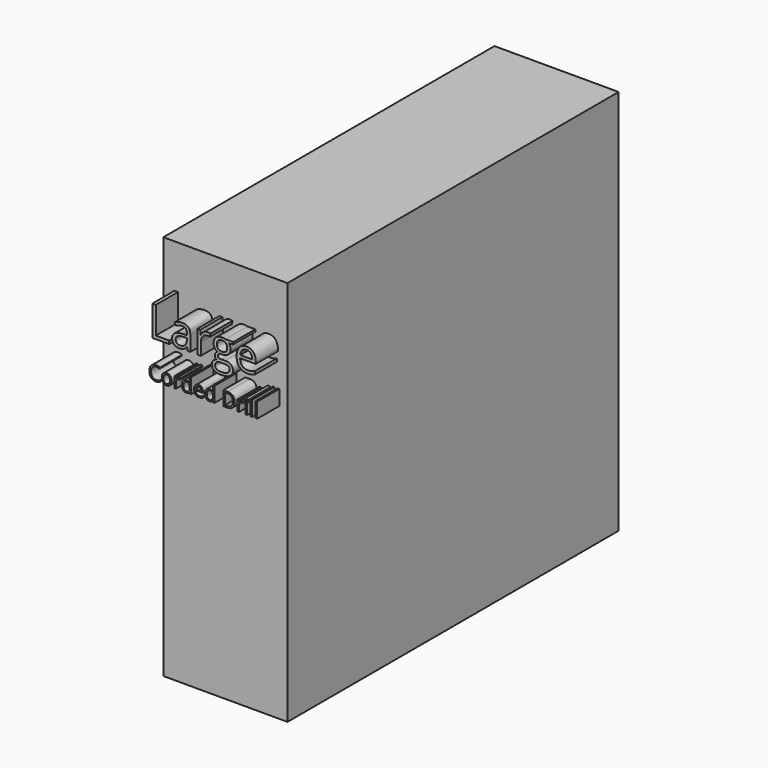
from build123d import *

# Parameters (mm, degrees)
F0_W           = 114.3
F0_H           = 355.6
F1_DEPTH       = 381
F2_TEXT_SIZE   = 39.0042588927
F2_TEXT_SIZE_2 = 18.2569631626
F3_DEPTH       = 25.4


# Not quite as in the source:
# - Text() gives the source's letters only with a copy of the font that has no kerning and outlines rounded to 1/6400 em; it was checked with that copy


with BuildPart() as f1:
    # F0 (on Front) → F1 (new body)
    with BuildSketch(Plane.XZ):
        Rectangle(F0_W, F0_H)
    extrude(amount=F1_DEPTH)

    # F2 (on face) → F3 (join)
    with BuildSketch(Plane.XZ.offset(381)):
        with Locations((-50.8, 109.8350980835)):
            Text('Large', F2_TEXT_SIZE, font='Open Sans', text_align=(TextAlign.LEFT, TextAlign.BOTTOM))
        with Locations((-50.8, 75.7488484937)):
            Text('Corded Drill', F2_TEXT_SIZE_2, font='Open Sans', text_align=(TextAlign.LEFT, TextAlign.BOTTOM))
    extrude(amount=F3_DEPTH)


solid = f1.part
